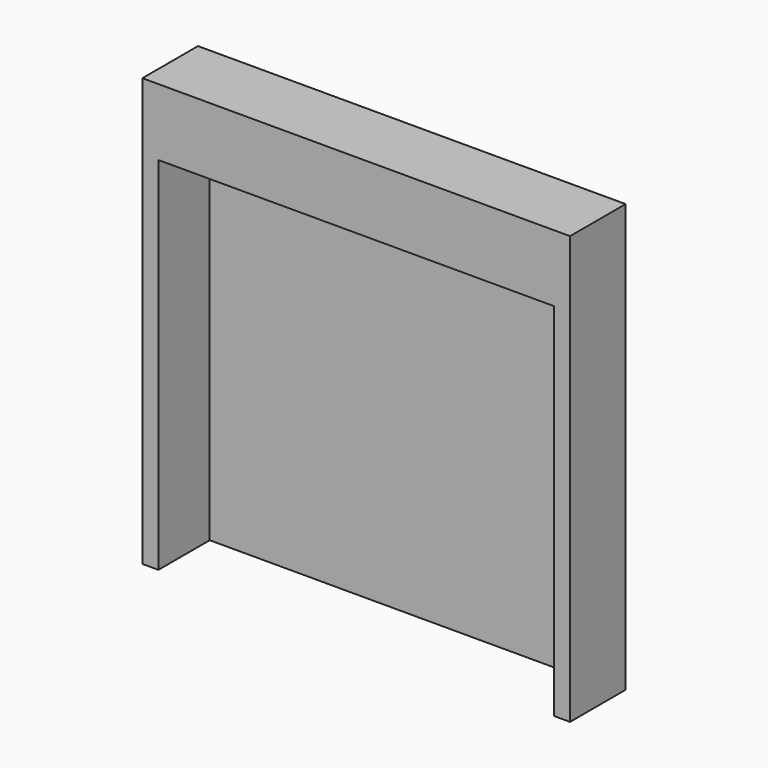
from build123d import *

# Parameters (mm, degrees)
F0_W     = 508
F0_H     = 508
F2_DEPTH = 6.35
F3_W     = 469.9
F3_H     = 79.375
F4_DEPTH = 76.2


with BuildPart() as f2:
    # F0 (on Front) → F2 (new body)
    with BuildSketch(Plane.XZ):
        with Locations((254, 254)):
            Rectangle(F0_W, F0_H)
    extrude(amount=F2_DEPTH)

    # F3 (on face) → F4 (join)
    with BuildSketch(Plane.XZ.offset(6.35)):
        Polygon((0, 508), (0, 0), (19.05, 0), (19.05, 428.625), (19.05, 508), align=None)
        with Locations((254, 468.3125)):
            Rectangle(F3_W, F3_H)
        Polygon((488.95, 508), (488.95, 428.625), (488.95, 0), (508, 0), (508, 508), align=None)
    extrude(amount=F4_DEPTH)


solid = f2.part
